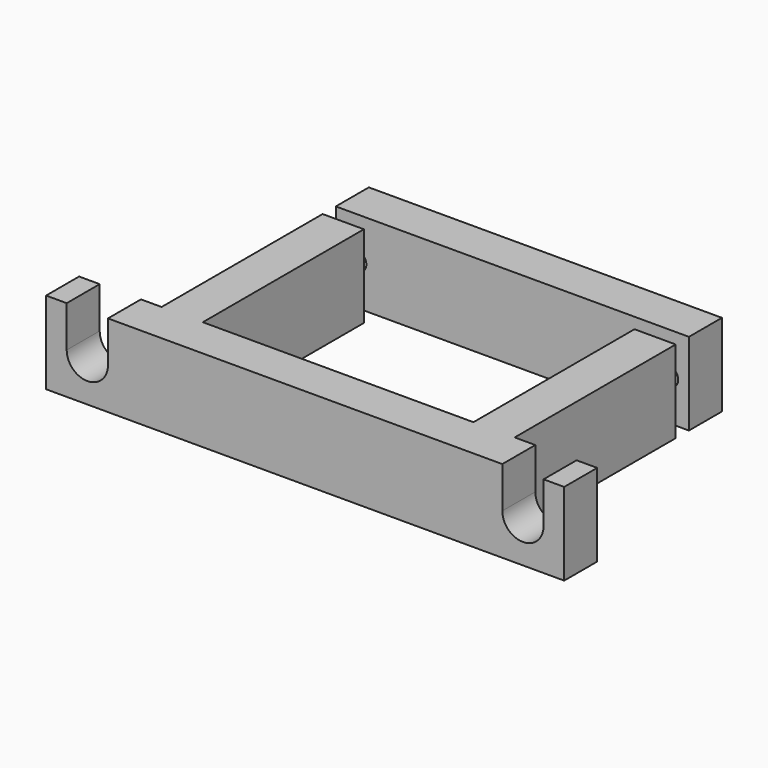
from build123d import *

# Parameters (mm, degrees)
F0_W     = 41.656
F0_H     = 33.528
F0_W_2   = 12.7
F0_H_2   = 6.35
F1_DEPTH = 12.7
F3_DEPTH = 6.351
F4_W     = 54.356
F4_H     = 2.54
F5_DEPTH = 12.701
F6_R     = 1.143
F7_DEPTH = 9.525
F8_R     = 1.524
F9_DEPTH = 6.35


# Not quite as in the source:
# - a pattern or mirror of a feature is missing from the dataset's text; its kind, count and spacing are read off the source's solid


with BuildPart() as f1:
    # F0 (on Top) → F1 (new body)
    with BuildSketch(Plane.XY):
        Polygon((27.178, -16.764), (27.178, 23.114), (-27.178, 23.114), (-27.178, -16.764), (-27.178, -23.114), (27.178, -23.114), align=None)
        Rectangle(F0_W, F0_H, mode=Mode.SUBTRACT)
        with Locations((33.528, -19.939)):
            Rectangle(F0_W_2, F0_H_2)
        with Locations((-33.528, -19.939)):
            Rectangle(F0_W_2, F0_H_2)
    extrude(amount=F1_DEPTH)

    # F2 (on face) → F3 (cut, through all)
    with BuildSketch(Plane(origin=(0, -16.764, 0), x_dir=(-1, 0, 0), z_dir=(0, 1, 0))):
        with BuildLine():
            Line((30.353, 12.7), (30.353, 6.35))
            ThreePointArc((30.353, 6.35), (33.528, 3.175), (36.703, 6.35))
            Line((36.703, 6.35), (36.703, 12.7))
            Line((36.703, 12.7), (30.353, 12.7))
        make_face()
    f3 = extrude(amount=-F3_DEPTH, mode=Mode.SUBTRACT)

    # F3_copies: F3 across plane
    add(f3.mirror(Plane(origin=(0, 0, 0), x_dir=(0, 0, 1), z_dir=(1, 0, 0))), mode=Mode.SUBTRACT)

    # F4 (on face) → F5 (cut, through all)
    with BuildSketch(Plane.XY.offset(12.7)):
        with Locations((0, 15.494)):
            Rectangle(F4_W, F4_H)
    extrude(amount=-F5_DEPTH, mode=Mode.SUBTRACT)

    # F6 (on face) → F7 (cut)
    with BuildSketch(Plane(origin=(0, 14.224, 0), x_dir=(-1, 0, 0), z_dir=(0, 1, 0))):
        with Locations((-24.003, 6.35)):
            Circle(F6_R)
    f7 = extrude(amount=-F7_DEPTH, mode=Mode.SUBTRACT)

    # F7_copies: F7 across plane
    add(f7.mirror(Plane(origin=(0, 0, 0), x_dir=(0, 0, -1), z_dir=(-1, 0, 0))), mode=Mode.SUBTRACT)

    # F8 (on face) → F9 (cut, through all)
    with BuildSketch(Plane(origin=(0, 23.114, 0), x_dir=(-1, 0, 0), z_dir=(0, 1, 0))):
        with Locations((-24.003, 6.35)):
            Circle(F8_R)
    f9 = extrude(amount=-F9_DEPTH, mode=Mode.SUBTRACT)

    # F9_copies: F9 across plane
    add(f9.mirror(Plane(origin=(0, 0, 0), x_dir=(0, 0, -1), z_dir=(-1, 0, 0))), mode=Mode.SUBTRACT)


solid = f1.part
